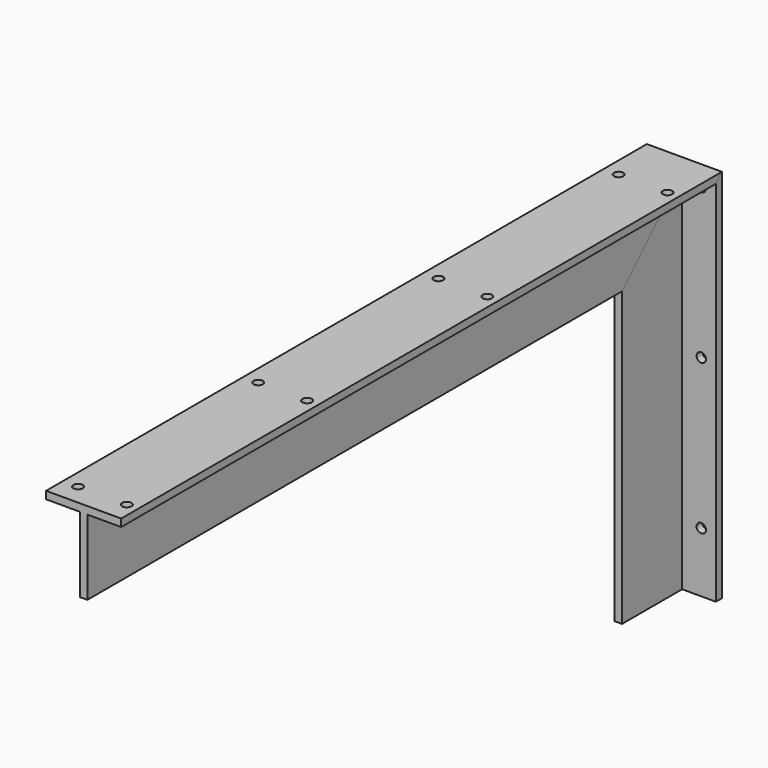
from build123d import *

# Parameters (mm, degrees)
F0_W     = 4
F0_H     = 40
F1_DEPTH = 200
F3_DEPTH = 51.9
F4_W     = 4
F4_H     = 40
F5_DEPTH = 200
F7_DEPTH = 41.7
F9_D     = 5
F11_D    = 5


with BuildPart() as f1:
    # F0 (on Front) → F1 (new body, symmetric)
    with BuildSketch(Plane.XZ):
        Polygon((18.5106403343, 24.7140824073), (-21.4893596657, 24.7140824073), (-21.4893596657, 20.7140824073), (-3.4893596657, 20.7140824073), (0.5106403343, 20.7140824073), (18.5106403343, 20.7140824073), align=None)
        with Locations((-1.4893596657, 0.7140824073)):
            Rectangle(F0_W, F0_H)
    extrude(amount=F1_DEPTH, both=True)

    # F2 (on face) → F3 (cut, symmetric)
    with BuildSketch(Plane(origin=(-21.4893596657, 0, 0), x_dir=(0, -1, 0), z_dir=(-1, 0, 0))):
        Polygon((-107.6650425279, -67.6208750648), (-196, 20.7140824073), (-200, 20.7140824073), (-200, -67.6208750648), align=None)
        Polygon((-196, 20.7140824073), (-200, 24.7140824073), (-200, 20.7140824073), align=None)
    extrude(amount=F3_DEPTH, both=True, mode=Mode.SUBTRACT)

    # F9 (through all)
    with Locations(Plane.XY.offset(24.7140824073)):
        with Locations((-13.4893596657, 171.2621307373), (12.5106403343, 171.2621307373), (12.5106403343, 51.2621307373), (-13.4893596657, 51.2621307373), (-13.4893596657, -68.7378692627), (12.5106403343, -68.7378692627), (-13.4893596657, -188.7378692627), (12.5106403343, -188.7378692627)):
            Hole(F9_D / 2)


with BuildPart() as f5:
    # F4 (on face) → F5 (new body)
    with BuildSketch(Plane.XY.offset(24.7140824073)):
        Polygon((18.5106403343, 200), (-21.4893596657, 200), (-21.4893596657, 196), (-3.4893596657, 196), (0.5106403343, 196), (18.5106403343, 196), align=None)
        with Locations((-1.4893596657, 176)):
            Rectangle(F4_W, F4_H)
    extrude(amount=-F5_DEPTH)

    # F6 (on face) → F7 (cut)
    with BuildSketch(Plane(origin=(-21.4893596657, 0, 0), x_dir=(0, -1, 0), z_dir=(-1, 0, 0))):
        Polygon((-196, 24.7140824073), (-196, 20.7140824073), (-144.8176057225, -30.4683118701), (-144.8176057225, 24.7140824073), align=None)
        Polygon((-196, 24.7140824073), (-200, 24.7140824073), (-196, 20.7140824073), align=None)
    extrude(amount=-F7_DEPTH, mode=Mode.SUBTRACT)

    # F11 (through all)
    with Locations(Plane(origin=(0, 200, 0), x_dir=(-1, 0, 0), z_dir=(0, 1, 0))):
        with Locations((-10.7106403343, 16.7140824073), (13.4893596657, 16.7140824073), (13.4893596657, -63.2859175927), (-10.7106403343, -63.2859175927), (-10.7106403343, -143.2859175927), (13.4893596657, -143.2859175927)):
            Hole(F11_D / 2)


solid = Compound([f1.part, f5.part])
